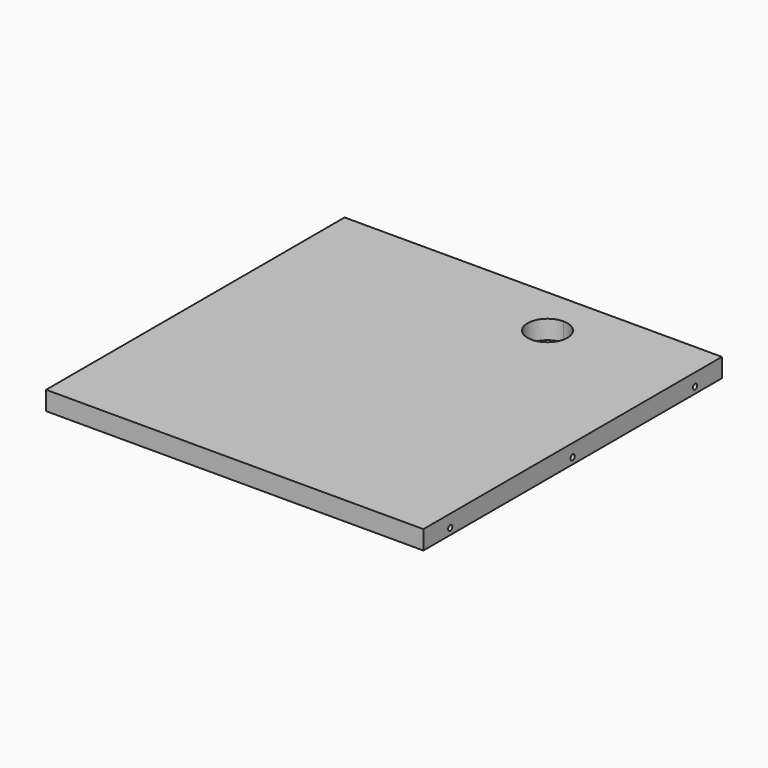
from build123d import *

# Parameters (mm, degrees)
F1_DEPTH  = 28.575
F3_D      = 15.0114
F3_DEPTH  = 14.224
F3_TIP    = 4.5098795482
F5_D      = 8.001
F5_DEPTH  = 25.4
F5_TIP    = 2.4037429064
F7_D      = 8.001
F7_DEPTH  = 25.4
F7_TIP    = 2.4037429064
F9_D      = 8.9916
F9_DEPTH  = 25.4
F9_TIP    = 2.701349171
F11_D     = 15.0114
F11_DEPTH = 14.224
F11_TIP   = 4.5098795482
F13_D     = 8.001
F13_DEPTH = 25.4
F13_TIP   = 2.4037429064


# Not quite as in the source:
# - a feature names something its author has since deleted; it is built from what else it names


with BuildPart() as f1:
    # F0 (on Top) → F1 (new body)
    with BuildSketch(Plane.XY):
        with BuildLine():
            Line((82.55, 236.5375), (82.55, 282.575))
            Line((82.55, 282.575), (-285.75, 282.575))
            Line((-285.75, 282.575), (-285.75, -282.575))
            Line((-285.75, -282.575), (285.75, -282.575))
            Line((285.75, -282.575), (285.75, 206.375))
            Line((285.75, 206.375), (112.7125, 206.375))
            ThreePointArc((112.7125, 206.375), (61.2218917125, 185.0468917125), (82.55, 236.5375))
        make_face()
        with BuildLine():
            Line((285.75, 206.375), (285.75, 282.575))
            Line((285.75, 282.575), (82.55, 282.575))
            Line((82.55, 282.575), (82.55, 236.5375))
            ThreePointArc((82.55, 236.5375), (103.8781082875, 227.7031082875), (112.7125, 206.375))
            Line((112.7125, 206.375), (285.75, 206.375))
        make_face()
    extrude(amount=F1_DEPTH)

    # F3
    with Locations(Plane(origin=(0, 0, 0), x_dir=(1, 0, 0), z_dir=(0, 0, -1))):
        with Locations((-261.874, 231.775), (261.874, 231.775), (-261.874, 0), (261.874, 0), (261.874, -231.775), (-261.874, -231.775)):
            Hole(F3_D / 2, depth=F3_DEPTH)
            with Locations((0, 0, -(F3_DEPTH + F3_TIP / 2))):  # 118° drill point
                Cone(0, F3_D / 2, F3_TIP, mode=Mode.SUBTRACT)

    # F5
    with Locations(Plane.YZ.offset(285.75)):
        with Locations((-231.775, 9.525), (0, 9.525), (231.775, 9.525)):
            Hole(F5_D / 2, depth=F5_DEPTH)
            with Locations((0, 0, -(F5_DEPTH + F5_TIP / 2))):  # 118° drill point
                Cone(0, F5_D / 2, F5_TIP, mode=Mode.SUBTRACT)

    # F7
    with Locations(Plane(origin=(-285.75, 0, 0), x_dir=(0, -1, 0), z_dir=(-1, 0, 0))):
        with Locations((0, 9.525), (231.775, 9.525), (-231.775, 9.525)):
            Hole(F7_D / 2, depth=F7_DEPTH)
            with Locations((0, 0, -(F7_DEPTH + F7_TIP / 2))):  # 118° drill point
                Cone(0, F7_D / 2, F7_TIP, mode=Mode.SUBTRACT)

    # F9
    with Locations(Plane(origin=(0, 0, 0), x_dir=(1, 0, 0), z_dir=(0, 0, -1))):
        with Locations((-228.6, -231.775), (-184.15, -231.775), (-184.15, -158.623), (-228.6, -158.623), (-228.6, 158.623), (-228.6, 231.775), (-184.15, 231.775), (-184.15, 158.623), (184.15, 231.775), (228.6, 231.775), (228.6, 158.623), (184.15, 158.623), (184.15, -158.623), (228.6, -158.623), (228.6, -231.775), (184.15, -231.775)):
            Hole(F9_D / 2, depth=F9_DEPTH)
            with Locations((0, 0, -(F9_DEPTH + F9_TIP / 2))):  # 118° drill point
                Cone(0, F9_D / 2, F9_TIP, mode=Mode.SUBTRACT)

    # F11
    with Locations(Plane(origin=(0, 0, 0), x_dir=(1, 0, 0), z_dir=(0, 0, -1))):
        with Locations((-234.95, -258.699), (234.95, -258.699)):
            Hole(F11_D / 2, depth=F11_DEPTH)
            with Locations((0, 0, -(F11_DEPTH + F11_TIP / 2))):  # 118° drill point
                Cone(0, F11_D / 2, F11_TIP, mode=Mode.SUBTRACT)

    # F13
    with Locations(Plane(origin=(0, 282.575, 0), x_dir=(-1, 0, 0), z_dir=(0, 1, 0))):
        with Locations((-234.95, 9.525), (234.95, 9.525)):
            Hole(F13_D / 2, depth=F13_DEPTH)
            with Locations((0, 0, -(F13_DEPTH + F13_TIP / 2))):  # 118° drill point
                Cone(0, F13_D / 2, F13_TIP, mode=Mode.SUBTRACT)


solid = f1.part
